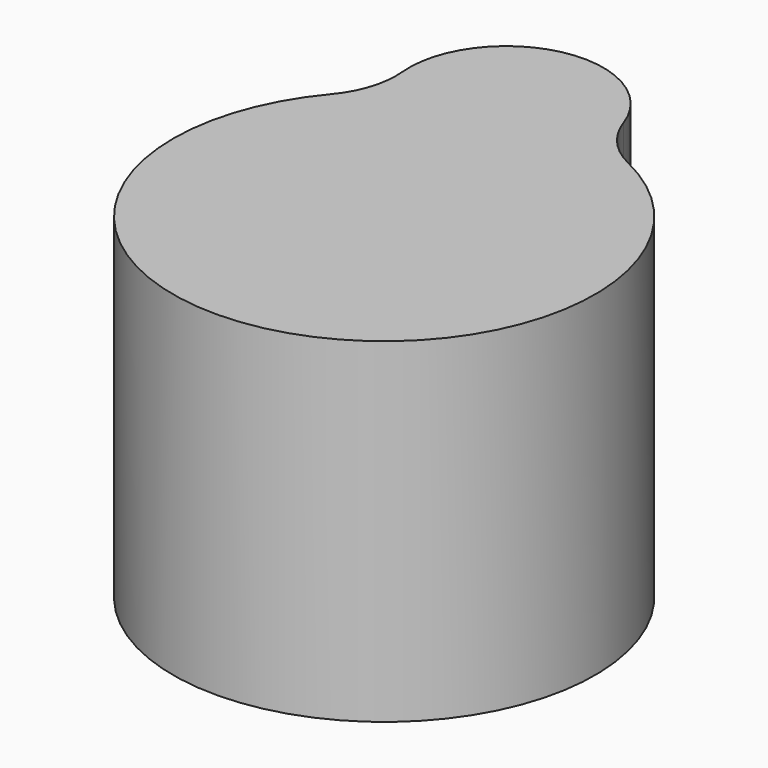
from build123d import *

# Parameters (mm, degrees)
F1_DEPTH = 58.42
F2_R     = 15.24
F3_R     = 6.8301694269
F4_DEPTH = 30.48


with BuildPart() as f1:
    # F0 (on Top) → F1 (new body)
    with BuildSketch(Plane.XY):
        with BuildLine():
            ThreePointArc((-22.9468365368, 28.7332625584), (-15.943079518, -33.1357193942), (36.7716967829, 0))
            ThreePointArc((36.7716967829, 0), (29.0432904816, 22.553158588), (9.1066714076, 35.6262013154))
            ThreePointArc((9.1066714076, 35.6262013154), (-7.7308275028, 35.9498538302), (-22.9468365368, 28.7332625584))
        make_face()
        with BuildLine():
            ThreePointArc((-22.9468365368, 28.7332625584), (-7.7308275028, 35.9498538302), (9.1066714076, 35.6262013154))
            ThreePointArc((9.1066714076, 35.6262013154), (-11.3815660909, 52.926499418), (-22.9468365368, 28.7332625584))
        make_face()
    extrude(amount=F1_DEPTH)

    # F2
    f2_edges = [f1.edges().sort_by_distance(p)[0] for p in [
        (9.106671, 35.626201, 29.21),
        (-22.946837, 28.733263, 29.21),
    ]]
    fillet(f2_edges, radius=F2_R)

    # F3 (on face) → F4 (join)
    with BuildSketch(Plane.XY.offset(58.42)):
        with Locations((-1.7507391749, 3.4323732834)):
            Circle(F3_R)
    extrude(amount=-F4_DEPTH)


solid = f1.part
